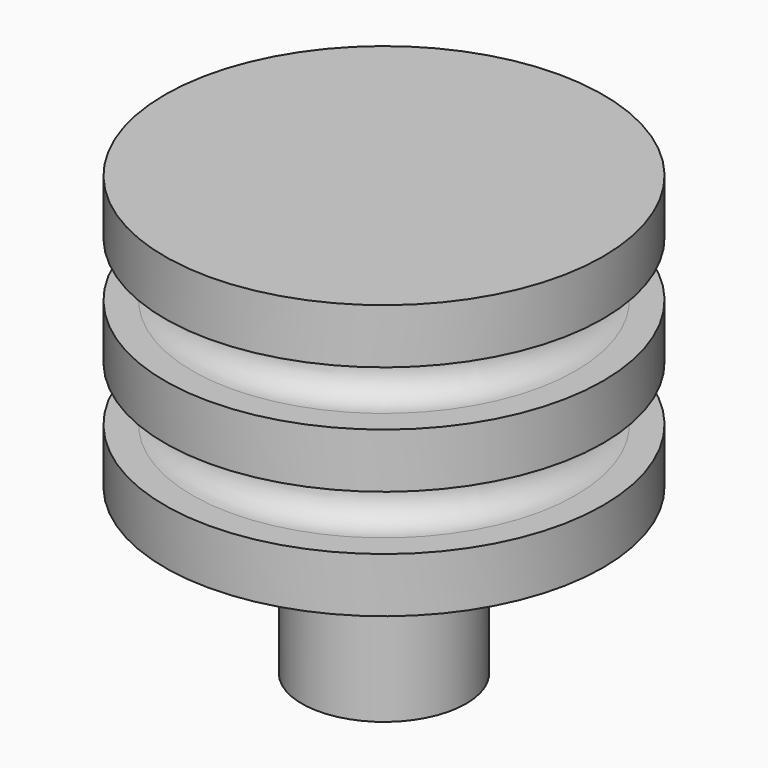
from build123d import *

# Parameters (mm, degrees)
F0_R     = 12.7
F0_R_2   = 4.7625
F1_DEPTH = 15.875
F3_DEPTH = 9.525
F4_W     = 3.175
F4_H     = 3.175
F6_R     = 1.58749


# Not quite as in the source:
# - a fillet or chamfer is up to 0.001 mm smaller than in the source, because OpenCascade refuses the exact size


with BuildPart() as f1:
    # F0 (on Top) → F1 (new body)
    with BuildSketch(Plane.XY):
        Circle(F0_R)
        Circle(F0_R_2, mode=Mode.SUBTRACT)
        Circle(F0_R_2)
    extrude(amount=F1_DEPTH)

    # F0 (on Top) → F3 (join)
    with BuildSketch(Plane.XY):
        Circle(F0_R_2)
    extrude(amount=-F3_DEPTH)

    # F4 (on Right) → F5 (revolve, cut)
    with BuildSketch(Plane.YZ):
        with Locations((11.1125, 4.7625)):
            Rectangle(F4_W, F4_H)
        with Locations((11.1125, 11.1125)):
            Rectangle(F4_W, F4_H)
    revolve(axis=Axis((0, 0, -0.284396112), (0, 0, 1)), mode=Mode.SUBTRACT)

    # F6 (radius 1.5875 in the source; OpenCascade refuses exactly that, so slightly less here)
    f6_edges = [f1.edges().sort_by_distance(p)[0] for p in [
        (0, -9.525, 3.175),
        (0, -9.525, 6.35),
        (0, -9.525, 9.525),
        (0, -9.525, 12.7),
    ]]
    fillet(f6_edges, radius=F6_R)


solid = f1.part
